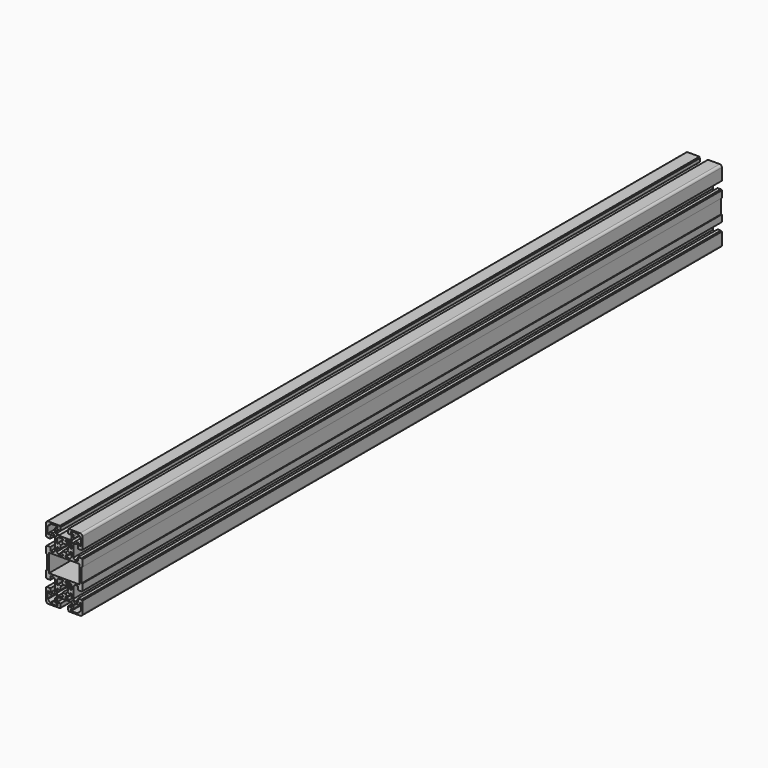
from build123d import *

# Parameters (mm, degrees)
F3_DEPTH = 1100


# Not quite as in the source:
# - ends of sketch curves that miss each other by under 0.0002 mm in the source are joined


with BuildPart() as f3:
    # F2 (on Front) → F3 (new body)
    with BuildSketch(Plane.XZ):
        with BuildLine():
            Line((21.000169, 12.449667), (21.000169, -0.000333))
            Line((21.000169, -0.000333), (24.000169, -0.000333))
            Line((24.000169, -0.000333), (24.000169, 9.999667))
            Line((24.000169, 9.999667), (25.000169, 9.999667))
            Line((25.000169, 9.999667), (25.000169, 19.199667))
            Line((25.000169, 19.199667), (23.500169, 19.199667))
            Line((23.500169, 19.199667), (23.500169, 19.999667))
            Line((23.500169, 19.999667), (19.000169, 19.999667))
            Line((19.000169, 19.999667), (19.000169, 14.949667))
            Line((19.000169, 14.949667), (14.800169, 14.949667))
            Line((14.800169, 14.949667), (12.500169, 17.249667))
            Line((12.500169, 17.249667), (12.500169, 32.749667))
            Line((12.500169, 32.749667), (14.800169, 35.049667))
            Line((14.800169, 35.049667), (19.000169, 35.049667))
            Line((19.000169, 35.049667), (19.000169, 29.999667))
            Line((19.000169, 29.999667), (23.500169, 29.999667))
            Line((23.500169, 29.999667), (23.500169, 30.799667))
            Line((23.500169, 30.799667), (25.000169, 30.799667))
            Line((25.000169, 30.799667), (25.000169, 46.999667))
            ThreePointArc((25.000169, 46.999667), (24.1214893436, 49.1209873436), (22.000169, 49.999667))
            Line((22.000169, 49.999667), (5.800169, 49.999667))
            Line((5.800169, 49.999667), (5.800169, 48.499667))
            Line((5.800169, 48.499667), (5.000169, 48.499667))
            Line((5.000169, 48.499667), (5.000169, 43.999667))
            Line((5.000169, 43.999667), (10.050169, 43.999667))
            Line((10.050169, 43.999667), (10.050169, 39.799667))
            Line((10.050169, 39.799667), (7.750169, 37.499667))
            Line((7.750169, 37.499667), (0.000169, 37.499667))
            Line((0.000169, 37.499667), (0.000169, 29.999667))
            ThreePointArc((0.000169, 29.999667), (1.0823669197, 29.8811470688), (2.1132600303, 29.531206065))
            Line((2.11326, 29.531206), (3.592424, 32.703283))
            Line((3.592424, 32.703283), (2.000169, 33.445764))
            Line((2.000169, 33.445764), (2.000169, 35.299667))
            Line((2.000169, 35.299667), (8.012449, 35.299667))
            Line((8.012449, 35.299667), (10.300169, 33.011947))
            Line((10.300169, 33.011947), (10.300169, 26.999667))
            Line((10.300169, 26.999667), (8.446266, 26.999667))
            Line((8.446266, 26.999667), (7.703785, 28.591922))
            Line((7.703785, 28.591922), (4.531708, 27.112758))
            ThreePointArc((4.531708065, 27.1127580303), (5.000169, 24.999667), (4.531708065, 22.8865759697))
            Line((4.531708, 22.886576), (7.703785, 21.407412))
            Line((7.703785, 21.407412), (8.446266, 22.999667))
            Line((8.446266, 22.999667), (10.300169, 22.999667))
            Line((10.300169, 22.999667), (10.300169, 16.987387))
            Line((10.300169, 16.987387), (8.012449, 14.699667))
            Line((8.012449, 14.699667), (2.000169, 14.699667))
            Line((2.000169, 14.699667), (2.000169, 16.55357))
            Line((2.000169, 16.55357), (3.592424, 17.296051))
            Line((3.592424, 17.296051), (2.11326, 20.468128))
            ThreePointArc((2.1132600303, 20.468127935), (1.0823669197, 20.1181869312), (0.000169, 19.999667))
            Line((0.000169, 19.999667), (0.000169, 12.449667))
            Line((0.000169, 12.449667), (21.000169, 12.449667))
        make_face()
        with BuildLine():
            Line((20.700169, 34.499667), (20.700169, 36.225912))
            ThreePointArc((20.700169, 36.225912), (20.1116343558, 37.41722678), (18.8078611265, 37.6737015332))
            ThreePointArc((18.8078611265, 37.6737015332), (17.1448966414, 37.5123048163), (15.5216018999, 37.9077967677))
            ThreePointArc((15.5216018999, 37.9077967677), (15.3464434299, 37.9269271737), (15.1907559656, 37.8444170344))
            Line((15.1907559656, 37.8444170344), (11.884862, 34.538523))
            Line((11.884862, 34.538523), (9.539025, 36.88436))
            Line((9.539025, 36.88436), (12.844919, 40.190254))
            ThreePointArc((12.844919, 40.190254), (12.9274291737, 40.3459414299), (12.9082991899, 40.5211000818))
            ThreePointArc((12.9082991899, 40.5211000818), (12.5128068163, 42.1443946414), (12.6742036668, 43.8073590903))
            ThreePointArc((12.6742036668, 43.8073590903), (12.41772878, 45.1111323558), (11.226414, 45.699667))
            Line((11.226414, 45.699667), (9.500169, 45.699667))
            Line((9.500169, 45.699667), (9.500169, 48.299667))
            Line((9.500169, 48.299667), (19.000169, 48.299667))
            Line((19.000169, 48.299667), (19.000169, 47.269363))
            ThreePointArc((19.000169, 47.269363), (21.0357029059, 46.0352009059), (22.2698650064, 43.999667002))
            Line((22.2698650064, 43.999667002), (23.300169, 43.999667))
            Line((23.300169, 43.999667), (23.300169, 34.499667))
            Line((23.300169, 34.499667), (20.700169, 34.499667))
        make_face(mode=Mode.SUBTRACT)
        with BuildLine():
            Line((-23.999831, -0.000333), (-20.999831, -0.000333))
            Line((-20.999831, -0.000333), (-20.999831, 12.449667))
            Line((-20.999831, 12.449667), (0.000169, 12.449667))
            Line((0.000169, 12.449667), (0.000169, 19.999667))
            ThreePointArc((0.000169, 19.999667), (-1.0820289197, 20.1181869312), (-2.1129220303, 20.468127935))
            Line((-2.112922, 20.468128), (-3.592086, 17.296051))
            Line((-3.592086, 17.296051), (-1.999831, 16.55357))
            Line((-1.999831, 16.55357), (-1.999831, 14.699667))
            Line((-1.999831, 14.699667), (-8.012111, 14.699667))
            Line((-8.012111, 14.699667), (-10.299831, 16.987387))
            Line((-10.299831, 16.987387), (-10.299831, 22.999667))
            Line((-10.299831, 22.999667), (-8.445928, 22.999667))
            Line((-8.445928, 22.999667), (-7.703447, 21.407412))
            Line((-7.703447, 21.407412), (-4.53137, 22.886576))
            ThreePointArc((-4.531370065, 22.8865759697), (-4.999831, 24.999667), (-4.531370065, 27.1127580303))
            Line((-4.53137, 27.112758), (-7.703447, 28.591922))
            Line((-7.703447, 28.591922), (-8.445928, 26.999667))
            Line((-8.445928, 26.999667), (-10.299831, 26.999667))
            Line((-10.299831, 26.999667), (-10.299831, 33.011947))
            Line((-10.299831, 33.011947), (-8.012111, 35.299667))
            Line((-8.012111, 35.299667), (-1.999831, 35.299667))
            Line((-1.999831, 35.299667), (-1.999831, 33.445764))
            Line((-1.999831, 33.445764), (-3.592086, 32.703283))
            Line((-3.592086, 32.703283), (-2.112922, 29.531206))
            ThreePointArc((-2.1129220303, 29.531206065), (-1.0820289197, 29.8811470688), (0.000169, 29.999667))
            Line((0.000169, 29.999667), (0.000169, 37.499667))
            Line((0.000169, 37.499667), (-7.749831, 37.499667))
            Line((-7.749831, 37.499667), (-10.049831, 39.799667))
            Line((-10.049831, 39.799667), (-10.049831, 43.999667))
            Line((-10.049831, 43.999667), (-4.999831, 43.999667))
            Line((-4.999831, 43.999667), (-4.999831, 48.499667))
            Line((-4.999831, 48.499667), (-5.799831, 48.499667))
            Line((-5.799831, 48.499667), (-5.799831, 49.999667))
            Line((-5.799831, 49.999667), (-21.999831, 49.999667))
            ThreePointArc((-21.999831, 49.999667), (-24.1211513436, 49.1209873436), (-24.999831, 46.999667))
            Line((-24.999831, 46.999667), (-24.999831, 30.799667))
            Line((-24.999831, 30.799667), (-23.499831, 30.799667))
            Line((-23.499831, 30.799667), (-23.499831, 29.999667))
            Line((-23.499831, 29.999667), (-18.999831, 29.999667))
            Line((-18.999831, 29.999667), (-18.999831, 35.049667))
            Line((-18.999831, 35.049667), (-14.799831, 35.049667))
            Line((-14.799831, 35.049667), (-12.499831, 32.749667))
            Line((-12.499831, 32.749667), (-12.499831, 17.249667))
            Line((-12.499831, 17.249667), (-14.799831, 14.949667))
            Line((-14.799831, 14.949667), (-18.999831, 14.949667))
            Line((-18.999831, 14.949667), (-18.999831, 19.999667))
            Line((-18.999831, 19.999667), (-23.499831, 19.999667))
            Line((-23.499831, 19.999667), (-23.499831, 19.199667))
            Line((-23.499831, 19.199667), (-24.999831, 19.199667))
            Line((-24.999831, 19.199667), (-24.999831, 9.999667))
            Line((-24.999831, 9.999667), (-23.999831, 9.999667))
            Line((-23.999831, 9.999667), (-23.999831, -0.000333))
        make_face()
        with BuildLine():
            ThreePointArc((-15.5212638999, 37.9077967677), (-17.1445586414, 37.5123048163), (-18.8075230903, 37.6737016668))
            ThreePointArc((-18.8075230903, 37.6737016668), (-20.1112963558, 37.41722678), (-20.699831, 36.225912))
            Line((-20.699831, 36.225912), (-20.699831, 34.499667))
            Line((-20.699831, 34.499667), (-23.299831, 34.499667))
            Line((-23.299831, 34.499667), (-23.299831, 43.999667))
            Line((-23.299831, 43.999667), (-22.269527, 43.999667))
            ThreePointArc((-22.269527, 43.999667), (-21.0353649059, 46.0352009059), (-18.999831002, 47.2693630064))
            Line((-18.999831002, 47.2693630064), (-18.999831, 48.299667))
            Line((-18.999831, 48.299667), (-9.499831, 48.299667))
            Line((-9.499831, 48.299667), (-9.499831, 45.699667))
            Line((-9.499831, 45.699667), (-11.226076, 45.699667))
            ThreePointArc((-11.226076, 45.699667), (-12.41739078, 45.1111323558), (-12.6738655332, 43.8073591265))
            ThreePointArc((-12.6738655332, 43.8073591265), (-12.5124688163, 42.1443946414), (-12.9079607677, 40.5210998999))
            ThreePointArc((-12.9079607677, 40.5210998999), (-12.9270911737, 40.3459414299), (-12.8445810344, 40.1902539656))
            Line((-12.8445810344, 40.1902539656), (-9.538687, 36.88436))
            Line((-9.538687, 36.88436), (-11.884524, 34.538523))
            Line((-11.884524, 34.538523), (-15.190418, 37.844417))
            ThreePointArc((-15.190418, 37.844417), (-15.3461054299, 37.9269271737), (-15.5212638999, 37.9077967677))
        make_face(mode=Mode.SUBTRACT)
        with BuildLine():
            Line((5.800169, -50.000333), (22.000169, -50.000333))
            ThreePointArc((22.000169, -50.000333), (24.1214893436, -49.1216533436), (25.000169, -47.000333))
            Line((25.000169, -47.000333), (25.000169, -30.800333))
            Line((25.000169, -30.800333), (23.500169, -30.800333))
            Line((23.500169, -30.800333), (23.500169, -30.000333))
            Line((23.500169, -30.000333), (19.000169, -30.000333))
            Line((19.000169, -30.000333), (19.000169, -35.050333))
            Line((19.000169, -35.050333), (14.800169, -35.050333))
            Line((14.800169, -35.050333), (12.500169, -32.750333))
            Line((12.500169, -32.750333), (12.500169, -17.250333))
            Line((12.500169, -17.250333), (14.800169, -14.950333))
            Line((14.800169, -14.950333), (19.000169, -14.950333))
            Line((19.000169, -14.950333), (19.000169, -20.000333))
            Line((19.000169, -20.000333), (23.500169, -20.000333))
            Line((23.500169, -20.000333), (23.500169, -19.200333))
            Line((23.500169, -19.200333), (25.000169, -19.200333))
            Line((25.000169, -19.200333), (25.000169, -10.000333))
            Line((25.000169, -10.000333), (24.000169, -10.000333))
            Line((24.000169, -10.000333), (24.000169, -0.000333))
            Line((24.000169, -0.000333), (21.000169, -0.000333))
            Line((21.000169, -0.000333), (21.000169, -12.450333))
            Line((21.000169, -12.450333), (0.000169, -12.450333))
            Line((0.000169, -12.450333), (0.000169, -20.000333))
            ThreePointArc((0.000169, -20.000333), (1.0823669197, -20.1188529312), (2.1132600303, -20.468793935))
            Line((2.11326, -20.468794), (3.592424, -17.296717))
            Line((3.592424, -17.296717), (2.000169, -16.554236))
            Line((2.000169, -16.554236), (2.000169, -14.700333))
            Line((2.000169, -14.700333), (8.012449, -14.700333))
            Line((8.012449, -14.700333), (10.300169, -16.988053))
            Line((10.300169, -16.988053), (10.300169, -23.000333))
            Line((10.300169, -23.000333), (8.446266, -23.000333))
            Line((8.446266, -23.000333), (7.703785, -21.408078))
            Line((7.703785, -21.408078), (4.531708, -22.887242))
            ThreePointArc((4.531708065, -22.8872419697), (5.000169, -25.000333), (4.531708065, -27.1134240303))
            Line((4.531708, -27.113424), (7.703785, -28.592588))
            Line((7.703785, -28.592588), (8.446266, -27.000333))
            Line((8.446266, -27.000333), (10.300169, -27.000333))
            Line((10.300169, -27.000333), (10.300169, -33.012613))
            Line((10.300169, -33.012613), (8.012449, -35.300333))
            Line((8.012449, -35.300333), (2.000169, -35.300333))
            Line((2.000169, -35.300333), (2.000169, -33.44643))
            Line((2.000169, -33.44643), (3.592424, -32.703949))
            Line((3.592424, -32.703949), (2.11326, -29.531872))
            ThreePointArc((2.1132600303, -29.531872065), (1.0823669197, -29.8818130688), (0.000169, -30.000333))
            Line((0.000169, -30.000333), (0.000169, -37.500333))
            Line((0.000169, -37.500333), (7.750169, -37.500333))
            Line((7.750169, -37.500333), (10.050169, -39.800333))
            Line((10.050169, -39.800333), (10.050169, -44.000333))
            Line((10.050169, -44.000333), (5.000169, -44.000333))
            Line((5.000169, -44.000333), (5.000169, -48.500333))
            Line((5.000169, -48.500333), (5.800169, -48.500333))
            Line((5.800169, -48.500333), (5.800169, -50.000333))
        make_face()
        with BuildLine():
            ThreePointArc((12.6742036668, -43.8080250903), (12.5128068163, -42.1450606414), (12.9082987677, -40.5217658999))
            ThreePointArc((12.9082987677, -40.5217658999), (12.9274291737, -40.3466074299), (12.8449190344, -40.1909199656))
            Line((12.8449190344, -40.1909199656), (9.539025, -36.885026))
            Line((9.539025, -36.885026), (11.884862, -34.539189))
            Line((11.884862, -34.539189), (15.190756, -37.845083))
            ThreePointArc((15.190756, -37.845083), (15.3464434299, -37.9275931737), (15.5216020818, -37.9084631899))
            ThreePointArc((15.5216020818, -37.9084631899), (17.1448966414, -37.5129708163), (18.8078610903, -37.6743676668))
            ThreePointArc((18.8078610903, -37.6743676668), (20.1116343558, -37.41789278), (20.700169, -36.226578))
            Line((20.700169, -36.226578), (20.700169, -34.500333))
            Line((20.700169, -34.500333), (23.300169, -34.500333))
            Line((23.300169, -34.500333), (23.300169, -44.000333))
            Line((23.300169, -44.000333), (22.269865, -44.000333))
            ThreePointArc((22.269865, -44.000333), (21.0357029059, -46.0358669059), (19.000169002, -47.2700290064))
            Line((19.000169002, -47.2700290064), (19.000169, -48.300333))
            Line((19.000169, -48.300333), (9.500169, -48.300333))
            Line((9.500169, -48.300333), (9.500169, -45.700333))
            Line((9.500169, -45.700333), (11.226414, -45.700333))
            ThreePointArc((11.226414, -45.700333), (12.41772878, -45.1117983558), (12.6742036668, -43.8080250903))
        make_face(mode=Mode.SUBTRACT)
        with BuildLine():
            Line((-7.749831, -37.500333), (0.000169, -37.500333))
            Line((0.000169, -37.500333), (0.000169, -30.000333))
            ThreePointArc((0.000169, -30.000333), (-1.0820289197, -29.8818130688), (-2.1129220303, -29.531872065))
            Line((-2.112922, -29.531872), (-3.592086, -32.703949))
            Line((-3.592086, -32.703949), (-1.999831, -33.44643))
            Line((-1.999831, -33.44643), (-1.999831, -35.300333))
            Line((-1.999831, -35.300333), (-8.012111, -35.300333))
            Line((-8.012111, -35.300333), (-10.299831, -33.012613))
            Line((-10.299831, -33.012613), (-10.299831, -27.000333))
            Line((-10.299831, -27.000333), (-8.445928, -27.000333))
            Line((-8.445928, -27.000333), (-7.703447, -28.592588))
            Line((-7.703447, -28.592588), (-4.53137, -27.113424))
            ThreePointArc((-4.531370065, -27.1134240303), (-4.999831, -25.000333), (-4.531370065, -22.8872419697))
            Line((-4.53137, -22.887242), (-7.703447, -21.408078))
            Line((-7.703447, -21.408078), (-8.445928, -23.000333))
            Line((-8.445928, -23.000333), (-10.299831, -23.000333))
            Line((-10.299831, -23.000333), (-10.299831, -16.988053))
            Line((-10.299831, -16.988053), (-8.012111, -14.700333))
            Line((-8.012111, -14.700333), (-1.999831, -14.700333))
            Line((-1.999831, -14.700333), (-1.999831, -16.554236))
            Line((-1.999831, -16.554236), (-3.592086, -17.296717))
            Line((-3.592086, -17.296717), (-2.112922, -20.468794))
            ThreePointArc((-2.1129220303, -20.468793935), (-1.0820289197, -20.1188529312), (0.000169, -20.000333))
            Line((0.000169, -20.000333), (0.000169, -12.450333))
            Line((0.000169, -12.450333), (-20.999831, -12.450333))
            Line((-20.999831, -12.450333), (-20.999831, -0.000333))
            Line((-20.999831, -0.000333), (-23.999831, -0.000333))
            Line((-23.999831, -0.000333), (-23.999831, -10.000333))
            Line((-23.999831, -10.000333), (-24.999831, -10.000333))
            Line((-24.999831, -10.000333), (-24.999831, -19.200333))
            Line((-24.999831, -19.200333), (-23.499831, -19.200333))
            Line((-23.499831, -19.200333), (-23.499831, -20.000333))
            Line((-23.499831, -20.000333), (-18.999831, -20.000333))
            Line((-18.999831, -20.000333), (-18.999831, -14.950333))
            Line((-18.999831, -14.950333), (-14.799831, -14.950333))
            Line((-14.799831, -14.950333), (-12.499831, -17.250333))
            Line((-12.499831, -17.250333), (-12.499831, -32.750333))
            Line((-12.499831, -32.750333), (-14.799831, -35.050333))
            Line((-14.799831, -35.050333), (-18.999831, -35.050333))
            Line((-18.999831, -35.050333), (-18.999831, -30.000333))
            Line((-18.999831, -30.000333), (-23.499831, -30.000333))
            Line((-23.499831, -30.000333), (-23.499831, -30.800333))
            Line((-23.499831, -30.800333), (-24.999831, -30.800333))
            Line((-24.999831, -30.800333), (-24.999831, -47.000333))
            ThreePointArc((-24.999831, -47.000333), (-24.1211513436, -49.1216533436), (-21.999831, -50.000333))
            Line((-21.999831, -50.000333), (-5.799831, -50.000333))
            Line((-5.799831, -50.000333), (-5.799831, -48.500333))
            Line((-5.799831, -48.500333), (-4.999831, -48.500333))
            Line((-4.999831, -48.500333), (-4.999831, -44.000333))
            Line((-4.999831, -44.000333), (-10.049831, -44.000333))
            Line((-10.049831, -44.000333), (-10.049831, -39.800333))
            Line((-10.049831, -39.800333), (-7.749831, -37.500333))
        make_face()
        with BuildLine():
            ThreePointArc((-12.9079607677, -40.5217658999), (-12.5124688163, -42.1450606414), (-12.6738656668, -43.8080250903))
            ThreePointArc((-12.6738656668, -43.8080250903), (-12.41739078, -45.1117983558), (-11.226076, -45.700333))
            Line((-11.226076, -45.700333), (-9.499831, -45.700333))
            Line((-9.499831, -45.700333), (-9.499831, -48.300333))
            Line((-9.499831, -48.300333), (-18.999831, -48.300333))
            Line((-18.999831, -48.300333), (-18.999831, -47.270029))
            ThreePointArc((-18.999831, -47.270029), (-21.0353649059, -46.0358669059), (-22.2695270064, -44.000333002))
            Line((-22.2695270064, -44.000333002), (-23.299831, -44.000333))
            Line((-23.299831, -44.000333), (-23.299831, -34.500333))
            Line((-23.299831, -34.500333), (-20.699831, -34.500333))
            Line((-20.699831, -34.500333), (-20.699831, -36.226578))
            ThreePointArc((-20.699831, -36.226578), (-20.1112963558, -37.41789278), (-18.8075231265, -37.6743675332))
            ThreePointArc((-18.8075231265, -37.6743675332), (-17.1445586414, -37.5129708163), (-15.5212638999, -37.9084627677))
            ThreePointArc((-15.5212638999, -37.9084627677), (-15.3461054299, -37.9275931737), (-15.1904179656, -37.8450830344))
            Line((-15.1904179656, -37.8450830344), (-11.884524, -34.539189))
            Line((-11.884524, -34.539189), (-9.538687, -36.885026))
            Line((-9.538687, -36.885026), (-12.844581, -40.19092))
            ThreePointArc((-12.844581, -40.19092), (-12.9270911737, -40.3466074299), (-12.9079607677, -40.5217658999))
        make_face(mode=Mode.SUBTRACT)
    extrude(amount=-F3_DEPTH)


solid = f3.part
